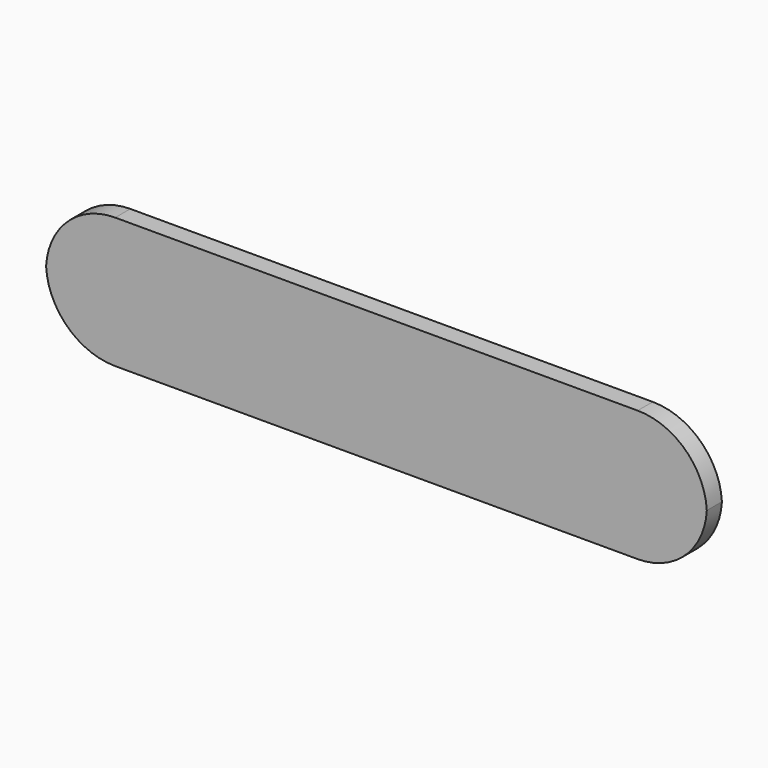
from build123d import *

# Parameters (mm, degrees)
F0_W        = 105
F0_H        = 20.7723644742
F1_DEPTH    = 3
F2_T1_DEPTH = 58


# Not quite as in the source:
# - a fillet or chamfer that OpenCascade refuses, or shapes differently, is made with other operations: its cross-section is extruded or revolved along the edge and cut away or added


with BuildPart() as f1:
    # F0 (on Front) → F1 (new body)
    with BuildSketch(Plane.XZ):
        Rectangle(F0_W, F0_H)
    extrude(amount=F1_DEPTH)

    # F2: fillet of radius 11 on 4 edges, made by hand

    # F2_s2 → F2_t1 (cut)
    with BuildSketch(Plane.XZ.offset(-27.5)):
        with BuildLine():
            ThreePointArc((-41.5, 10.3861822371), (-49.2781745931, 7.1643568302), (-52.5, -0.6138177629))
            Line((-52.5, -0.6138177629), (-52.5, 10.3861822371))
            Line((-52.5, 10.3861822371), (-41.5, 10.3861822371))
        make_face()
        with BuildLine():
            ThreePointArc((-52.5, 0.6138177629), (-49.2781745931, -7.1643568302), (-41.5, -10.3861822371))
            Line((-41.5, -10.3861822371), (-52.5, -10.3861822371))
            Line((-52.5, -10.3861822371), (-52.5, 0.6138177629))
        make_face()
        with BuildLine():
            ThreePointArc((52.5, -0.6138177629), (49.2781745931, 7.1643568302), (41.5, 10.3861822371))
            Line((41.5, 10.3861822371), (52.5, 10.3861822371))
            Line((52.5, 10.3861822371), (52.5, -0.6138177629))
        make_face()
        with BuildLine():
            ThreePointArc((52.5, 0.6138177629), (49.2781745931, -7.1643568302), (41.5, -10.3861822371))
            Line((41.5, -10.3861822371), (52.5, -10.3861822371))
            Line((52.5, -10.3861822371), (52.5, 0.6138177629))
        make_face()
    extrude(amount=F2_T1_DEPTH, mode=Mode.SUBTRACT)


solid = f1.part
